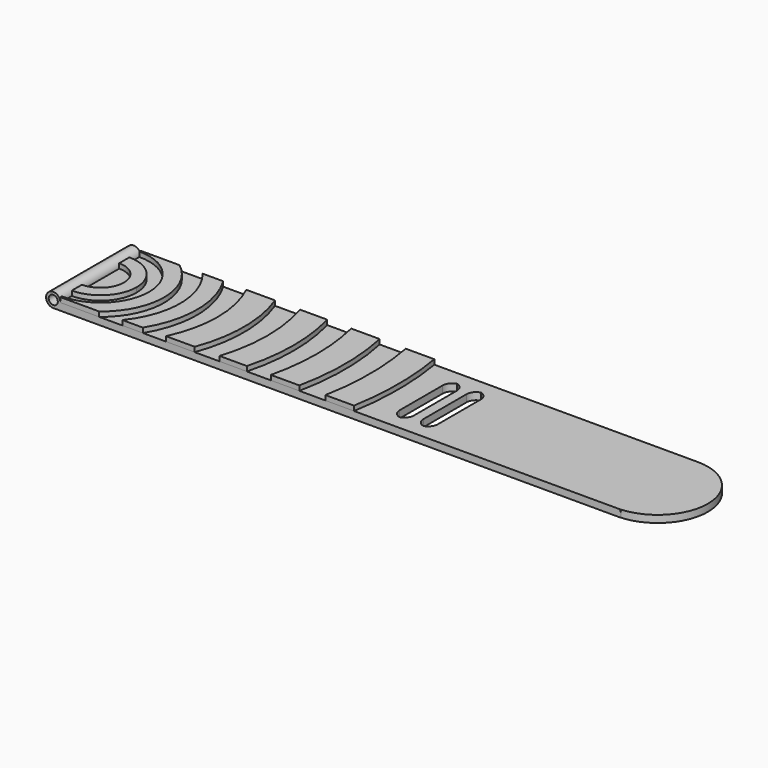
from build123d import *

# Parameters (mm, degrees)
F1_DEPTH    = 21
F3_DEPTH    = 1.5
F4_R        = 0.95
F5_DEPTH    = 25.4
F6_W        = 2.9805600643
F6_H        = 15.2461954355
F7_DEPTH    = 25.4
F8_T1_DEPTH = 1.5
F9_T1_DEPTH = 1.5
F11_DEPTH   = 1


# Not quite as in the source:
# - a fillet or chamfer that OpenCascade refuses, or shapes differently, is made with other operations: its cross-section is extruded or revolved along the edge and cut away or added


with BuildPart() as f1:
    # F0 (on Front) → F1 (new body)
    with BuildSketch(Plane.XZ):
        with BuildLine():
            ThreePointArc((0, -1.5), (1.0606601718, -1.0606601718), (1.5, 0))
            ThreePointArc((1.5, 0), (-1.0606601718, 1.0606601718), (0, -1.5))
        make_face()
        with BuildLine():
            Line((118, 0), (1.5, 0))
            ThreePointArc((1.5, 0), (1.0606601718, -1.0606601718), (0, -1.5))
            Line((0, -1.5), (118, -1.5))
            ThreePointArc((118, -1.5), (118.75, -0.75), (118, 0))
        make_face()
    extrude(amount=-F1_DEPTH)

    # F2 (on face) → F3 (join)
    with BuildSketch(Plane(origin=(0, 0, -1.5), x_dir=(1, 0, 0), z_dir=(0, 0, -1))):
        with BuildLine():
            Line((118, 0), (118, -21))
            ThreePointArc((118, -21), (128.5, -10.5), (118, 0))
        make_face()
    extrude(amount=-F3_DEPTH)

    # F4 (on face) → F5 (cut)
    with BuildSketch(Plane.XZ):
        Circle(F4_R)
    extrude(amount=-F5_DEPTH, mode=Mode.SUBTRACT)

    # F6 (on face) → F7 (cut)
    with BuildSketch(Plane.XY):
        with Locations((70.0291599035, 10.4999999497)):
            Rectangle(F6_W, F6_H)
        with Locations((75.0097199678, 10.5)):
            Rectangle(F6_W, F6_H)
    extrude(amount=-F7_DEPTH, mode=Mode.SUBTRACT)

    # F8: fillet of radius 2 on 4 edges, made by hand

    # F8_s2 → F8_t1 (join)
    with BuildSketch(Plane.XY.offset(-1.5)):
        with BuildLine():
            ThreePointArc((70.5388798714, 2.8769022319), (69.124666309, 3.4626886696), (68.5388798714, 4.8769022319))
            Line((68.5388798714, 4.8769022319), (68.5388798714, 2.8769022319))
            Line((68.5388798714, 2.8769022319), (70.5388798714, 2.8769022319))
        make_face()
        with BuildLine():
            ThreePointArc((70.5388798714, 18.1230976675), (69.124666309, 17.5373112298), (68.5388798714, 16.1230976675))
            Line((68.5388798714, 16.1230976675), (68.5388798714, 18.1230976675))
            Line((68.5388798714, 18.1230976675), (70.5388798714, 18.1230976675))
        make_face()
        with BuildLine():
            ThreePointArc((71.5194399357, 16.1230976675), (70.9336534981, 17.5373112298), (69.5194399357, 18.1230976675))
            Line((69.5194399357, 18.1230976675), (71.5194399357, 18.1230976675))
            Line((71.5194399357, 18.1230976675), (71.5194399357, 16.1230976675))
        make_face()
        with BuildLine():
            ThreePointArc((69.5194399357, 2.8769022319), (70.9336534981, 3.4626886696), (71.5194399357, 4.8769022319))
            Line((71.5194399357, 4.8769022319), (71.5194399357, 2.8769022319))
            Line((71.5194399357, 2.8769022319), (69.5194399357, 2.8769022319))
        make_face()
    extrude(amount=F8_T1_DEPTH)

    # F9: fillet of radius 2 on 4 edges, made by hand

    # F9_s2 → F9_t1 (join)
    with BuildSketch(Plane.XY.offset(-1.5)):
        with BuildLine():
            ThreePointArc((75.5194399357, 18.1230977178), (74.1052263733, 17.5373112801), (73.5194399357, 16.1230977178))
            Line((73.5194399357, 16.1230977178), (73.5194399357, 18.1230977178))
            Line((73.5194399357, 18.1230977178), (75.5194399357, 18.1230977178))
        make_face()
        with BuildLine():
            ThreePointArc((73.5194399357, 4.8769022822), (74.1052263733, 3.4626887199), (75.5194399357, 2.8769022822))
            Line((75.5194399357, 2.8769022822), (73.5194399357, 2.8769022822))
            Line((73.5194399357, 2.8769022822), (73.5194399357, 4.8769022822))
        make_face()
        with BuildLine():
            ThreePointArc((76.5, 4.8769022822), (75.9142135624, 3.4626887199), (74.5, 2.8769022822))
            Line((74.5, 2.8769022822), (76.5, 2.8769022822))
            Line((76.5, 2.8769022822), (76.5, 4.8769022822))
        make_face()
        with BuildLine():
            ThreePointArc((76.5, 16.1230977178), (75.9142135624, 17.5373112801), (74.5, 18.1230977178))
            Line((74.5, 18.1230977178), (76.5, 18.1230977178))
            Line((76.5, 18.1230977178), (76.5, 16.1230977178))
        make_face()
    extrude(amount=F9_T1_DEPTH)


with BuildPart() as f11:
    # F10 (on face) → F11 (new body)
    with BuildSketch(Plane.XY):
        with BuildLine():
            Line((1.5, 18.0205481217), (1.5, 15.3751391684))
            ThreePointArc((1.5, 15.3751391684), (4.9472439652, 13.9472439652), (6.3751391684, 10.5))
            ThreePointArc((6.3751391684, 10.5), (4.9472439652, 7.0527560348), (1.5, 5.6248608316))
            Line((1.5, 5.6248608316), (1.5, 2.9794518783))
            ThreePointArc((1.5, 2.9794518783), (6.8178305751, 5.1821694249), (9.0205481217, 10.5))
            ThreePointArc((9.0205481217, 10.5), (6.8178305751, 15.8178305751), (1.5, 18.0205481217))
        make_face()
    extrude(amount=F11_DEPTH)


with BuildPart() as f11b:
    # F10 (on face) → F11, piece 2 (new body)
    with BuildSketch(Plane.XY):
        with BuildLine():
            Line((1.5, 21), (1.5, 20.6492265591))
            ThreePointArc((1.5, 20.6492265591), (8.6765869237, 17.6765869237), (11.6492265591, 10.5))
            ThreePointArc((11.6492265591, 10.5), (8.6765869237, 3.3234130763), (1.5, 0.3507734409))
            Line((1.5, 0.3507734409), (1.5, 0))
            Line((1.5, 0), (9.6176613001, 0))
            ThreePointArc((9.6176613001, 0), (14.7720166133, 10.5), (9.6176613001, 21))
            Line((9.6176613001, 21), (1.5, 21))
        make_face()
    extrude(amount=F11_DEPTH)


with BuildPart() as f11c:
    # F10 (on face) → F11, piece 3 (new body)
    with BuildSketch(Plane.XY):
        with BuildLine():
            Line((18.7453661335, 21), (14.4430249836, 21))
            ThreePointArc((14.4430249836, 21), (18.1664902042, 10.5), (14.4430249836, 0))
            Line((14.4430249836, 0), (18.7453661335, 0))
            ThreePointArc((18.7453661335, 0), (21.6904099284, 10.5), (18.7453661335, 21))
        make_face()
    extrude(amount=F11_DEPTH)


with BuildPart() as f11d:
    # F10 (on face) → F11, piece 4 (new body)
    with BuildSketch(Plane.XY):
        with BuildLine():
            Line((29.5774242132, 21), (23.5667478281, 21))
            ThreePointArc((23.5667478281, 21), (25.9374990477, 10.5), (23.5667478281, 0))
            Line((23.5667478281, 0), (29.5774242132, 0))
            ThreePointArc((29.5774242132, 0), (31.4765199856, 10.5), (29.5774242132, 21))
        make_face()
    extrude(amount=F11_DEPTH)


with BuildPart() as f11e:
    # F10 (on face) → F11, piece 5 (new body)
    with BuildSketch(Plane.XY):
        with BuildLine():
            Line((40.4886008324, 21), (34.7911855171, 21))
            ThreePointArc((34.7911855171, 21), (36.4077789774, 10.5), (34.7911855171, 0))
            Line((34.7911855171, 0), (40.4886008324, 0))
            ThreePointArc((40.4886008324, 0), (41.8777289464, 10.5), (40.4886008324, 21))
        make_face()
    extrude(amount=F11_DEPTH)


with BuildPart() as f11f:
    # F10 (on face) → F11, piece 6 (new body)
    with BuildSketch(Plane.XY):
        with BuildLine():
            Line((51.4633184784, 21), (45.5065769526, 21))
            ThreePointArc((45.5065769526, 21), (46.741892258, 10.5), (45.5065769526, 0))
            Line((45.5065769526, 0), (51.4633184784, 0))
            ThreePointArc((51.4633184784, 0), (52.5547078473, 10.5), (51.4633184784, 21))
        make_face()
    extrude(amount=F11_DEPTH)


with BuildPart() as f11g:
    # F10 (on face) → F11, piece 7 (new body)
    with BuildSketch(Plane.XY):
        with BuildLine():
            Line((62.8874615739, 21), (56.9114878139, 21))
            ThreePointArc((56.9114878139, 21), (57.897544111, 10.5), (56.9114878139, 0))
            Line((56.9114878139, 0), (62.8874615739, 0))
            ThreePointArc((62.8874615739, 0), (63.7789726833, 10.5), (62.8874615739, 21))
        make_face()
    extrude(amount=F11_DEPTH)


solid = Compound([f1.part, f11.part, f11b.part, f11c.part, f11d.part, f11e.part, f11f.part, f11g.part])
